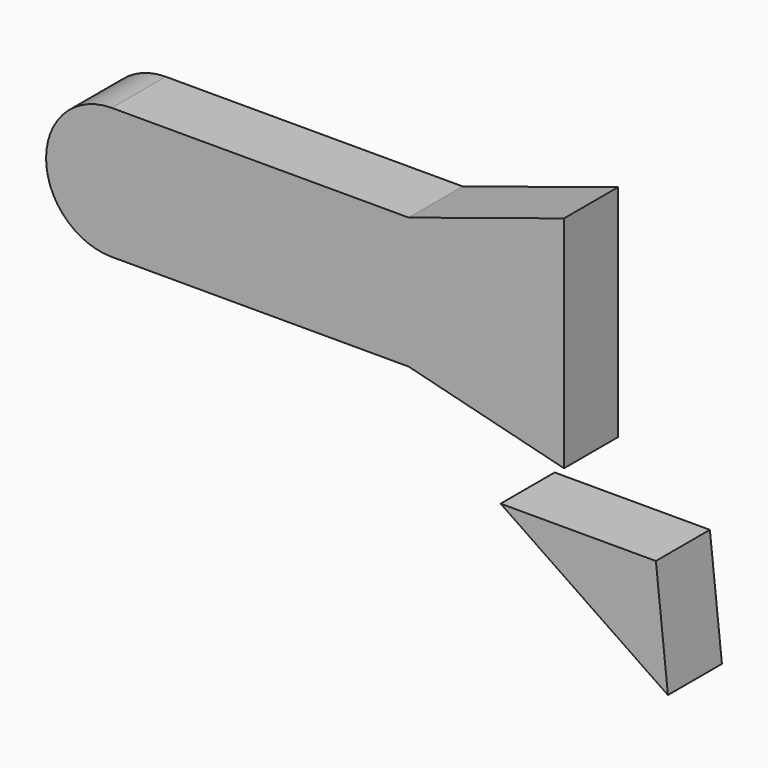
from build123d import *

# Parameters (mm, degrees)
F0_W     = 111.7699816823
F0_H     = 49.370786408
F1_DEPTH = 25.4
F2_DEPTH = 25.4
F4_DEPTH = 25.4


# Not quite as in the source:
# - the program builds the solid bodies; features that only make, move or delete a surface that nothing else refers to are left out


with BuildPart() as f1:
    # F0 (on Front) → F1 (new body)
    with BuildSketch(Plane.XZ):
        with Locations((-136.135738343, 27.4491094751)):
            Rectangle(F0_W, F0_H)
        with BuildLine():
            Line((-192.0207291842, 2.7637162711), (-192.0207291842, 52.1345026791))
            ThreePointArc((-192.0207291842, 52.1345026791), (-216.7061223881, 27.4491094751), (-192.0207291842, 2.7637162711))
        make_face()
        Polygon((-21.8198485672, 70.8749219775), (-80.2507475019, 52.1345026791), (-80.2507475019, 2.7637162711), (-21.8198485672, -11.922063306), align=None)
    extrude(amount=F1_DEPTH)

    # F0 (on Front) → F2 (join)
    with BuildSketch(Plane.XZ):
        with Locations((-136.135738343, 27.4491094751)):
            Rectangle(F0_W, F0_H)
        with BuildLine():
            Line((-192.0207291842, 2.7637162711), (-192.0207291842, 52.1345026791))
            ThreePointArc((-192.0207291842, 52.1345026791), (-216.7061223881, 27.4491094751), (-192.0207291842, 2.7637162711))
        make_face()
        Polygon((-21.8198485672, 70.8749219775), (-80.2507475019, 52.1345026791), (-80.2507475019, 2.7637162711), (-21.8198485672, -11.922063306), align=None)
    extrude(amount=F2_DEPTH)


with BuildPart() as f4:
    # F3 (on Front) → F4 (new body)
    with BuildSketch(Plane.XZ):
        Polygon((12.7544817491, -31.3732413198), (-45.6655182509, -31.3732413198), (17.282307836, -74.3151927301), align=None)
    extrude(amount=F4_DEPTH)


solid = Compound([f1.part, f4.part])
